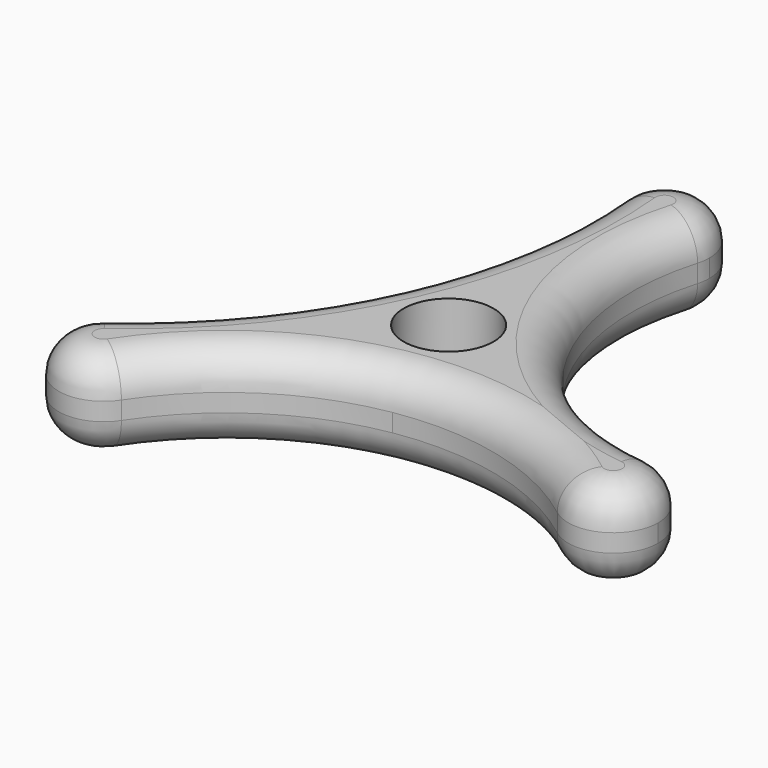
from build123d import *

# Parameters (mm, degrees)
F0_R         = 6.35
F1_DEPTH     = 12.7
F2_T2_ANGLE  = 99.446116479
F2_T4_ANGLE  = 59.2916827944
F2_T6_ANGLE  = 201.7148311049
F2_T8_ANGLE  = 200.3212768017
F2_T10_ANGLE = 94.2324188496
F2_T12_ANGLE = 210.9341102164
F2_T14_ANGLE = 94.2324188496
F2_T16_ANGLE = 210.9341102164
F2_T18_ANGLE = 200.3212768017
F2_T20_ANGLE = 59.2916827944
F2_T22_ANGLE = 201.7148311049
F2_T24_ANGLE = 99.446116479


# Not quite as in the source:
# - a fillet or chamfer that OpenCascade refuses, or shapes differently, is made with other operations: its cross-section is extruded or revolved along the edge and cut away or added


with BuildPart() as f1:
    # F0 (on Top) → F1 (new body)
    with BuildSketch(Plane.XY):
        with BuildLine():
            ThreePointArc((-23.0979636954, -28.8973481426), (-12.2116587197, -18.0861984821), (2.0883176929, -12.527127732))
            ThreePointArc((2.0883176929, -12.527127732), (-10.0506029407, -7.7637220795), (-11.5934607492, 5.1847534038))
            ThreePointArc((-11.5934607492, 5.1847534038), (-20.2173700121, -8.8847131705), (-32.1537121721, -20.2796873478))
            ThreePointArc((-32.1537121721, -20.2796873478), (-25.5280345903, -19.7355993147), (-22.0480633142, -25.4))
            ThreePointArc((-22.0480633142, -25.4), (-22.3161995958, -27.2257693475), (-23.0979636954, -28.8973481426))
        make_face()
        with BuildLine():
            ThreePointArc((10.5830984733, 7.0205431916), (12.1592629425, 3.6663775985), (12.7, 0))
            ThreePointArc((12.7, 0), (9.6905013983, -8.2087869171), (2.0883176929, -12.527127732))
            ThreePointArc((2.0883176929, -12.527127732), (17.4183090092, -13.1467749254), (31.2229657331, -19.8418514101))
            ThreePointArc((31.2229657331, -19.8418514101), (29.2220209534, -12.4165925694), (35.8447458338, -8.5079145294))
            ThreePointArc((35.8447458338, -8.5079145294), (21.5024747262, -3.5278630909), (10.5830984733, 7.0205431916))
        make_face()
        with BuildLine():
            ThreePointArc((-11.5934607492, 5.1847534038), (-1.0477304131, 12.6567081416), (10.5830984733, 7.0205431916))
            ThreePointArc((10.5830984733, 7.0205431916), (5.1104904876, 21.1821889646), (6.0989820006, 36.3322560831))
            ThreePointArc((6.0989820006, 36.3322560831), (-0.5872613397, 31.7772138958), (-6.320221624, 37.4857536138))
            ThreePointArc((-6.320221624, 37.4857536138), (-6.8559724512, 20.992280129), (-11.5934607492, 5.1847534038))
        make_face()
        with BuildLine():
            ThreePointArc((2.0883176929, -12.527127732), (9.6905013983, -8.2087869171), (12.7, 0))
            ThreePointArc((12.7, 0), (12.1592629425, 3.6663775985), (10.5830984733, 7.0205431916))
            ThreePointArc((10.5830984733, 7.0205431916), (-1.0477304131, 12.6567081416), (-11.5934607492, 5.1847534038))
            ThreePointArc((-11.5934607492, 5.1847534038), (-10.0506029407, -7.7637220795), (2.0883176929, -12.527127732))
        make_face()
        Circle(F0_R, mode=Mode.SUBTRACT)
        with BuildLine():
            ThreePointArc((-32.1537121721, -20.2796873478), (-32.7755456308, -30.0000161487), (-23.0979636954, -28.8973481426))
            ThreePointArc((-23.0979636954, -28.8973481426), (-22.3161995958, -27.2257693475), (-22.0480633142, -25.4))
            ThreePointArc((-22.0480633142, -25.4), (-25.5280345903, -19.7355993147), (-32.1537121721, -20.2796873478))
        make_face()
        with BuildLine():
            ThreePointArc((41.4519366858, -14.8143187798), (39.8474260225, -10.5949786709), (35.8447458338, -8.5079145294))
            ThreePointArc((35.8447458338, -8.5079145294), (29.2220209534, -12.4165925694), (31.2229657331, -19.8418514101))
            ThreePointArc((31.2229657331, -19.8418514101), (37.9029217313, -20.5131768035), (41.4519366858, -14.8143187798))
        make_face()
        with BuildLine():
            ThreePointArc((-6.320221624, 37.4857536138), (-0.5872613397, 31.7772138958), (6.0989820006, 36.3322560831))
            ThreePointArc((6.0989820006, 36.3322560831), (6.2869323085, 37.2072614336), (6.35, 38.1))
            ThreePointArc((6.35, 38.1), (-0.3074838917, 44.442551037), (-6.320221624, 37.4857536138))
        make_face()
    extrude(amount=F1_DEPTH)

    # F2: fillet of radius 5.08 on 12 edges, made by hand

    # F2_s1 → F2_t2 (revolve, cut)
    with BuildSketch(Plane(origin=(36.3426576492, -4.2806736606, 0), x_dir=(0, 0, 1), z_dir=(0.9931345276, -0.1169778186, 0))):
        with BuildLine():
            ThreePointArc((7.62, 4.2564635014), (11.2121024484, 5.744361053), (12.7, 9.3364635014))
            Line((12.7, 9.3364635014), (12.7, 4.2564635014))
            Line((12.7, 4.2564635014), (7.62, 4.2564635014))
        make_face()
    revolve(axis=Axis((39.9699722036, 26.5150051248, 12.7), (0, 0, -1)), revolution_arc=F2_T2_ANGLE, mode=Mode.SUBTRACT)

    # F2_s3 → F2_t4 (revolve, cut)
    with BuildSketch(Plane(origin=(-3.6681952371, 37.7434973641, 0), x_dir=(0, 0, 1), z_dir=(-0.0967317144, 0.995310492, 0))):
        with BuildLine():
            ThreePointArc((7.62, -2.6645216828), (11.2121024484, -1.1766241312), (12.7, 2.4154783172))
            Line((12.7, 2.4154783172), (12.7, -2.6645216828))
            Line((12.7, -2.6645216828), (7.62, -2.6645216828))
        make_face()
    revolve(axis=Axis((-69.9851672009, 31.2983182556, 12.7), (0, 0, -1)), revolution_arc=F2_T4_ANGLE, mode=Mode.SUBTRACT)

    # F2_s5 → F2_t6 (revolve, cut)
    with BuildSketch(Plane(origin=(10.1871858245, 35.1473210497, 0), x_dir=(0, 0, 1), z_dir=(-0.2783848688, -0.9604696064, 0))):
        with BuildLine():
            ThreePointArc((7.62, 4.2564635014), (11.2121024484, 5.744361053), (12.7, 9.3364635014))
            Line((12.7, 9.3364635014), (12.7, 4.2564635014))
            Line((12.7, 4.2564635014), (7.62, 4.2564635014))
        make_face()
    revolve(axis=Axis((0, 38.1, 12.7), (0, 0, 1)), revolution_arc=F2_T6_ANGLE, mode=Mode.SUBTRACT)

    # F2_s7 → F2_t8 (revolve, cut)
    with BuildSketch(Plane(origin=(-30.5778054296, -22.4282202745, 0), x_dir=(0, 0, 1), z_dir=(0.8063484492, 0.591440765, 0))):
        with BuildLine():
            ThreePointArc((7.62, -2.6645216828), (11.2121024484, -1.1766241312), (12.7, 2.4154783172))
            Line((12.7, 2.4154783172), (12.7, -2.6645216828))
            Line((12.7, -2.6645216828), (7.62, -2.6645216828))
        make_face()
    revolve(axis=Axis((-28.3980633142, -25.4, 12.7), (0, 0, 1)), revolution_arc=F2_T8_ANGLE, mode=Mode.SUBTRACT)

    # F2_s9 → F2_t10 (revolve, cut)
    with BuildSketch(Plane(origin=(-20.2906858047, -30.7497714597, 0), x_dir=(0, 0, 1), z_dir=(-0.550763487, -0.8346613573, 0))):
        with BuildLine():
            ThreePointArc((5.08, 3.3633735001), (1.4878975516, 4.8512710517), (0, 8.4433735001))
            Line((0, 8.4433735001), (0, 3.3633735001))
            Line((0, 3.3633735001), (5.08, 3.3633735001))
        make_face()
    revolve(axis=Axis((8.2675580223, -49.5943457482, 0), (0, 0, -1)), revolution_arc=F2_T10_ANGLE, mode=Mode.SUBTRACT)

    # F2_s11 → F2_t12 (revolve, cut)
    with BuildSketch(Plane(origin=(29.1684101252, -22.5047600746, 0), x_dir=(0, 0, 1), z_dir=(-0.7917374221, 0.6108615673, 0))):
        with BuildLine():
            ThreePointArc((5.08, 3.3633735001), (1.4878975516, 4.8512710517), (0, 8.4433735001))
            Line((0, 8.4433735001), (0, 3.3633735001))
            Line((0, 3.3633735001), (5.08, 3.3633735001))
        make_face()
    revolve(axis=Axis((35.1019366858, -14.8143187798, 0), (0, 0, 1)), revolution_arc=F2_T12_ANGLE, mode=Mode.SUBTRACT)

    # F2_s13 → F2_t14 (revolve, cut)
    with BuildSketch(Plane(origin=(-20.2906858047, -30.7497714597, 0), x_dir=(0, 0, 1), z_dir=(-0.550763487, -0.8346613573, 0))):
        with BuildLine():
            ThreePointArc((7.62, 3.3633735001), (11.2121024484, 4.8512710517), (12.7, 8.4433735001))
            Line((12.7, 8.4433735001), (12.7, 3.3633735001))
            Line((12.7, 3.3633735001), (7.62, 3.3633735001))
        make_face()
    revolve(axis=Axis((8.2675580223, -49.5943457482, 12.7), (0, 0, -1)), revolution_arc=F2_T14_ANGLE, mode=Mode.SUBTRACT)

    # F2_s15 → F2_t16 (revolve, cut)
    with BuildSketch(Plane(origin=(29.1684101252, -22.5047600746, 0), x_dir=(0, 0, 1), z_dir=(-0.7917374221, 0.6108615673, 0))):
        with BuildLine():
            ThreePointArc((7.62, 3.3633735001), (11.2121024484, 4.8512710517), (12.7, 8.4433735001))
            Line((12.7, 8.4433735001), (12.7, 3.3633735001))
            Line((12.7, 3.3633735001), (7.62, 3.3633735001))
        make_face()
    revolve(axis=Axis((35.1019366858, -14.8143187798, 12.7), (0, 0, 1)), revolution_arc=F2_T16_ANGLE, mode=Mode.SUBTRACT)

    # F2_s17 → F2_t18 (revolve, cut)
    with BuildSketch(Plane(origin=(-30.5778054296, -22.4282202745, 0), x_dir=(0, 0, 1), z_dir=(0.8063484492, 0.591440765, 0))):
        with BuildLine():
            ThreePointArc((5.08, -2.6645216828), (1.4878975516, -1.1766241312), (0, 2.4154783172))
            Line((0, 2.4154783172), (0, -2.6645216828))
            Line((0, -2.6645216828), (5.08, -2.6645216828))
        make_face()
    revolve(axis=Axis((-28.3980633142, -25.4, 0), (0, 0, 1)), revolution_arc=F2_T18_ANGLE, mode=Mode.SUBTRACT)

    # F2_s19 → F2_t20 (revolve, cut)
    with BuildSketch(Plane(origin=(-3.6681952371, 37.7434973641, 0), x_dir=(0, 0, 1), z_dir=(-0.0967317144, 0.995310492, 0))):
        with BuildLine():
            ThreePointArc((5.08, -2.6645216828), (1.4878975516, -1.1766241312), (0, 2.4154783172))
            Line((0, 2.4154783172), (0, -2.6645216828))
            Line((0, -2.6645216828), (5.08, -2.6645216828))
        make_face()
    revolve(axis=Axis((-69.9851672009, 31.2983182556, 0), (0, 0, -1)), revolution_arc=F2_T20_ANGLE, mode=Mode.SUBTRACT)

    # F2_s21 → F2_t22 (revolve, cut)
    with BuildSketch(Plane(origin=(10.1871858245, 35.1473210497, 0), x_dir=(0, 0, 1), z_dir=(-0.2783848688, -0.9604696064, 0))):
        with BuildLine():
            ThreePointArc((5.08, 4.2564635014), (1.4878975516, 5.744361053), (0, 9.3364635014))
            Line((0, 9.3364635014), (0, 4.2564635014))
            Line((0, 4.2564635014), (5.08, 4.2564635014))
        make_face()
    revolve(axis=Axis((0, 38.1, 0), (0, 0, 1)), revolution_arc=F2_T22_ANGLE, mode=Mode.SUBTRACT)

    # F2_s23 → F2_t24 (revolve, cut)
    with BuildSketch(Plane(origin=(36.3426576492, -4.2806736606, 0), x_dir=(0, 0, 1), z_dir=(0.9931345276, -0.1169778186, 0))):
        with BuildLine():
            ThreePointArc((5.08, 4.2564635014), (1.4878975516, 5.744361053), (0, 9.3364635014))
            Line((0, 9.3364635014), (0, 4.2564635014))
            Line((0, 4.2564635014), (5.08, 4.2564635014))
        make_face()
    revolve(axis=Axis((39.9699722036, 26.5150051248, 0), (0, 0, -1)), revolution_arc=F2_T24_ANGLE, mode=Mode.SUBTRACT)


solid = f1.part
